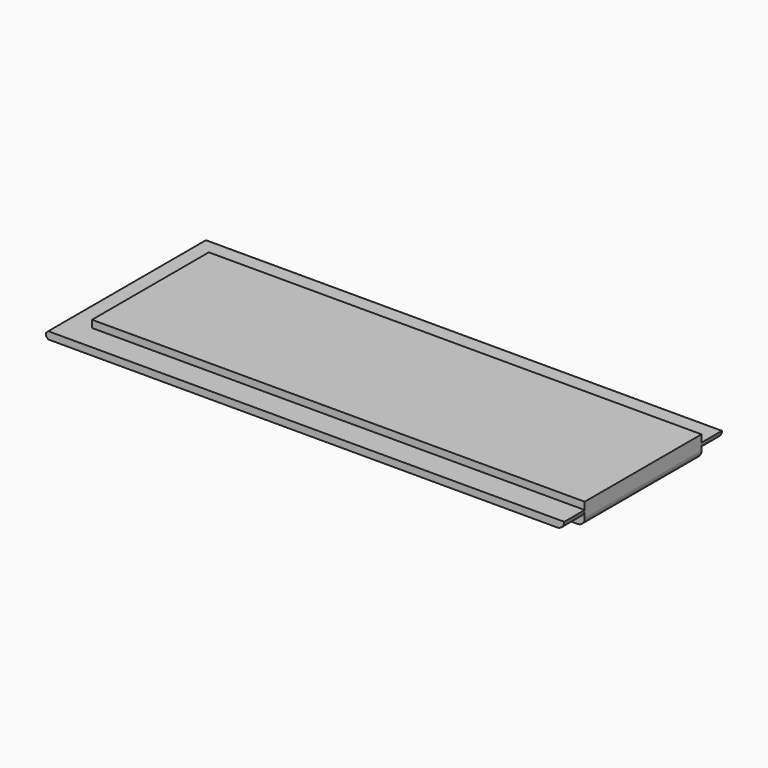
from build123d import *

# Parameters (mm, degrees)
F0_W         = 67.5
F0_H         = 20
F1_DEPTH     = 1
F2_W         = 71
F2_H         = 27
F3_DEPTH     = 1
F4_W         = 67.5
F4_H         = 20
F5_DEPTH     = 1
F6_R         = 0.99999
F7_R         = 1
F8_W         = 2
F8_H         = 15
F9_DEPTH     = 4
F10_T1_DEPTH = 26.4948974279
F11_SIZE     = 0.3


# Not quite as in the source:
# - a fillet or chamfer that OpenCascade refuses, or shapes differently, is made with other operations: its cross-section is extruded or revolved along the edge and cut away or added
# - a fillet or chamfer is up to 0.001 mm smaller than in the source, because OpenCascade refuses the exact size


with BuildPart() as f1:
    # F0 (on Top) → F1 (new body)
    with BuildSketch(Plane.XY):
        with Locations((-4.0991377383, -20.9536040443)):
            Rectangle(F0_W, F0_H)
    extrude(amount=F1_DEPTH)

    # F2 (on face) → F3 (join)
    with BuildSketch(Plane.XY.offset(1)):
        with Locations((-5.8491377383, -20.9536040443)):
            Rectangle(F2_W, F2_H)
    extrude(amount=F3_DEPTH)

    # F4 (on face) → F5 (join)
    with BuildSketch(Plane.XY.offset(2)):
        with Locations((-4.0991377383, -20.9536040443)):
            Rectangle(F4_W, F4_H)
    extrude(amount=F5_DEPTH)

    # F6 (radius 1 in the source; OpenCascade refuses exactly that, so slightly less here)
    f6_edges = [f1.edges().sort_by_distance(p)[0] for p in [
        (29.650862, -9.203604, 1),
        (29.650862, -32.703604, 1),
    ]]
    fillet(f6_edges, radius=F6_R)

    # F7
    f7_edges = [f1.edges().sort_by_distance(p)[0] for p in [
        (29.650862, -20.953604, 0),
    ]]
    fillet(f7_edges, radius=F7_R)

    # F8 (on face) → F9 (join)
    with BuildSketch(Plane(origin=(0, 0, 0), x_dir=(1, 0, 0), z_dir=(0, 0, -1))):
        with Locations((14.6508622617, 20.9536040443)):
            Rectangle(F8_W, F8_H)
    extrude(amount=F9_DEPTH)

    # F10: fillet of radius 5 on 2 edges, made by hand

    # F10_s2 → F10_t1 (cut)
    with BuildSketch(Plane.YZ.offset(1.4034135477)):
        with BuildLine():
            ThreePointArc((-28.4536040443, 0), (-26.7169022189, -2.8729833462), (-23.5546245587, -4))
            Line((-23.5546245587, -4), (-28.4536040443, -4))
            Line((-28.4536040443, -4), (-28.4536040443, 0))
        make_face()
        with BuildLine():
            ThreePointArc((-13.4536040443, 0), (-15.1903058697, -2.8729833462), (-18.3525835299, -4))
            Line((-18.3525835299, -4), (-13.4536040443, -4))
            Line((-13.4536040443, -4), (-13.4536040443, 0))
        make_face()
    extrude(amount=F10_T1_DEPTH, mode=Mode.SUBTRACT)

    # F11
    f11_edges = [f1.edges().sort_by_distance(p)[0] for p in [
        (-41.349138, -20.953604, 2),
        (-41.349138, -20.953604, 1),
    ]]
    chamfer(f11_edges, length=F11_SIZE)


solid = f1.part
